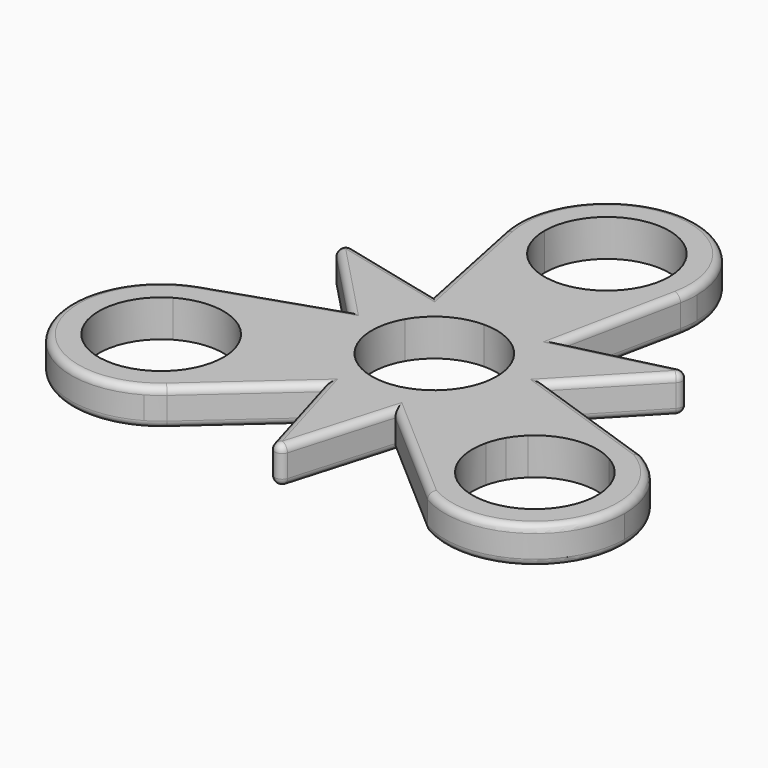
from build123d import *

# Parameters (mm, degrees)
F1_DEPTH      = 6.5278
F2_T3_ANGLE   = 203.1236625431
F2_T6_DEPTH   = 24.7868945093
F2_T10_DEPTH  = 28.7612147001
F2_T14_DEPTH  = 28.7612147001
F2_T18_DEPTH  = 24.7868937804
F2_T22_ANGLE  = 203.1236592361
F2_T25_DEPTH  = 24.7868960458
F2_T29_DEPTH  = 28.7612147001
F2_T33_DEPTH  = 28.8510148795
F2_T37_DEPTH  = 33.4056274337
F2_T41_ANGLE  = 202.9551687841
F2_T44_DEPTH  = 33.4056274337
F2_T48_DEPTH  = 28.8510148795
F2_T52_DEPTH  = 28.7612147001
F2_T56_DEPTH  = 24.7868944005
F2_T60_DEPTH  = 24.7868945093
F2_T64_ANGLE  = 203.1236625431
F2_T67_DEPTH  = 24.7868944005
F2_T71_DEPTH  = 28.7612147001
F2_T75_DEPTH  = 28.8510148795
F2_T79_DEPTH  = 33.4056274337
F2_T83_DEPTH  = 33.4056274337
F2_T87_ANGLE  = 202.9551687841
F2_T90_DEPTH  = 28.8510148795
F2_T94_DEPTH  = 28.7612147001
F2_T98_DEPTH  = 24.7868960458
F2_T102_ANGLE = 203.1236592361
F2_T105_DEPTH = 28.7612147001
F2_T109_DEPTH = 28.7612147001
F2_T113_DEPTH = 24.7868937804
F2_T118_DEPTH = 24.7868945093
F2_T122_DEPTH = 28.7612147001
F2_T128_DEPTH = 28.7612147001
F2_T132_DEPTH = 24.7868937804
F2_T138_DEPTH = 24.7868960458
F2_T142_DEPTH = 28.7612147001
F2_T148_DEPTH = 28.8510148795
F2_T152_DEPTH = 33.4056274337
F2_T158_DEPTH = 33.4056274337
F2_T162_DEPTH = 28.8510148795
F2_T168_DEPTH = 28.7612147001
F2_T172_DEPTH = 24.7868944005
F2_T178_DEPTH = 24.7868945093
F2_T182_DEPTH = 28.7612147001
F2_T188_DEPTH = 28.7612147001
F2_T192_DEPTH = 24.7868944005
F2_T198_DEPTH = 33.4056274337
F2_T202_DEPTH = 28.8510148795
F2_T208_DEPTH = 28.8510148795
F2_T212_DEPTH = 33.4056274337
F2_T218_DEPTH = 24.7868960458
F2_T222_DEPTH = 28.7612147001
F2_T228_DEPTH = 28.7612147001
F2_T232_DEPTH = 24.7868937804
F3_T1_DEPTH   = 3.9878
F3_T6_DEPTH   = 1.27
F3_T12_DEPTH  = 1.27
F3_T18_DEPTH  = 1.27
F3_T24_DEPTH  = 1.27
F3_T30_DEPTH  = 1.27
F3_T36_DEPTH  = 1.27


# Not quite as in the source:
# - a fillet or chamfer that OpenCascade refuses, or shapes differently, is made with other operations: its cross-section is extruded or revolved along the edge and cut away or added
# - a feature names something its author has since deleted; it is built from what else it names


with BuildPart() as f1:
    # F0 (on Top) → F1 (new body)
    with BuildSketch(Plane.XY):
        with BuildLine():
            ThreePointArc((-9.5357191185, 5.50545), (-5.50545, 9.5357191185), (0, 11.0109))
            Line((0, 11.0109), (-7.397765026, 12.8133048875))
            Line((-7.397765026, 12.8133048875), (-9.5357191185, 5.50545))
        make_face()
        with BuildLine():
            Line((-32.9955678842, 19.05), (-13.7481532851, 7.9375))
            ThreePointArc((-13.7481532851, 7.9375), (-12.4088537844, 9.9013116685), (-10.7913433943, 11.6431324285))
            Line((-10.7913433943, 11.6431324285), (-11.2213112334, 13.7448806198))
            Line((-11.2213112334, 13.7448806198), (-32.9955678842, 19.05))
        make_face()
        with BuildLine():
            ThreePointArc((-15.4789201598, 3.5240113062), (-14.7792143279, 5.7957267749), (-13.7481532851, 7.9375))
            Line((-13.7481532851, 7.9375), (-32.9955678842, 19.05))
            Line((-32.9955678842, 19.05), (-17.5140714054, 2.8455002819))
            Line((-17.5140714054, 2.8455002819), (-15.4789201598, 3.5240113062))
        make_face()
        with BuildLine():
            Line((-15.4789201598, 3.5240113062), (-9.5357191185, 5.50545))
            Line((-9.5357191185, 5.50545), (-13.7481532851, 7.9375))
            ThreePointArc((-13.7481532851, 7.9375), (-14.7792143279, 5.7957267749), (-15.4789201598, 3.5240113062))
        make_face()
        with BuildLine():
            Line((-14.795530052, 0), (-9.5357191185, 5.50545))
            Line((-9.5357191185, 5.50545), (-15.4789201598, 3.5240113062))
            ThreePointArc((-15.4789201598, 3.5240113062), (-15.7054057137, 2.3142723193), (-15.8374924179, 1.0906231763))
            Line((-15.8374924179, 1.0906231763), (-14.795530052, 0))
        make_face()
        with BuildLine():
            ThreePointArc((-9.5357191185, -5.50545), (-11.0109, 0), (-9.5357191185, 5.50545))
            Line((-9.5357191185, 5.50545), (-14.795530052, 0))
            Line((-14.795530052, 0), (-9.5357191185, -5.50545))
        make_face()
        with BuildLine():
            Line((-13.7481532851, 7.9375), (-9.5357191185, 5.50545))
            Line((-9.5357191185, 5.50545), (-10.7913433943, 11.6431324285))
            ThreePointArc((-10.7913433943, 11.6431324285), (-12.4088537844, 9.9013116685), (-13.7481532851, 7.9375))
        make_face()
        with BuildLine():
            Line((-11.2213112334, 13.7448806198), (-10.7913433943, 11.6431324285))
            ThreePointArc((-10.7913433943, 11.6431324285), (-9.8569214766, 12.4441441652), (-8.8632535856, 13.170359178))
            Line((-8.8632535856, 13.170359178), (-11.2213112334, 13.7448806198))
        make_face()
        with BuildLine():
            Line((-10.7913433943, 11.6431324285), (-9.5357191185, 5.50545))
            Line((-9.5357191185, 5.50545), (-7.397765026, 12.8133048875))
            Line((-7.397765026, 12.8133048875), (-8.8632535856, 13.170359178))
            ThreePointArc((-8.8632535856, 13.170359178), (-9.8569214766, 12.4441441652), (-10.7913433943, 11.6431324285))
        make_face()
        with BuildLine():
            ThreePointArc((-8.8632535856, 13.170359178), (-7.9375, 13.7481532851), (-6.9742388323, 14.2609823543))
            Line((-6.9742388323, 14.2609823543), (-4.4574811793, 22.863645891))
            ThreePointArc((-4.4574811793, 22.863645891), (-11.6804109204, 27.3490174528), (-15.5528801368, 34.9182482102))
            Line((-15.5528801368, 34.9182482102), (-11.2213112334, 13.7448806198))
            Line((-11.2213112334, 13.7448806198), (-8.8632535856, 13.170359178))
        make_face()
        with BuildLine():
            ThreePointArc((-6.9742388323, 14.2609823543), (-3.5792827581, 15.4662328942), (0, 15.875))
            Line((0, 15.875), (0, 22.225))
            ThreePointArc((0, 22.225), (-2.2514998911, 22.3854725416), (-4.4574811793, 22.863645891))
            Line((-4.4574811793, 22.863645891), (-6.9742388323, 14.2609823543))
        make_face()
        with BuildLine():
            Line((0, 15.875), (0, 11.0109))
            Line((0, 11.0109), (7.397765026, 12.8133048875))
            Line((7.397765026, 12.8133048875), (6.9742388323, 14.2609823543))
            ThreePointArc((6.9742388323, 14.2609823543), (3.5792827581, 15.4662328942), (0, 15.875))
        make_face()
        with BuildLine():
            Line((-7.397765026, 12.8133048875), (0, 11.0109))
            Line((0, 11.0109), (0, 15.875))
            ThreePointArc((0, 15.875), (-3.5792827581, 15.4662328942), (-6.9742388323, 14.2609823543))
            Line((-6.9742388323, 14.2609823543), (-7.397765026, 12.8133048875))
        make_face()
        with BuildLine():
            Line((-8.8632535856, 13.170359178), (-7.397765026, 12.8133048875))
            Line((-7.397765026, 12.8133048875), (-6.9742388323, 14.2609823543))
            ThreePointArc((-6.9742388323, 14.2609823543), (-7.9375, 13.7481532851), (-8.8632535856, 13.170359178))
        make_face()
        with BuildLine():
            ThreePointArc((-15.8374924179, 1.0906231763), (-15.7054057137, 2.3142723193), (-15.4789201598, 3.5240113062))
            Line((-15.4789201598, 3.5240113062), (-17.5140714054, 2.8455002819))
            Line((-17.5140714054, 2.8455002819), (-15.8374924179, 1.0906231763))
        make_face()
        with BuildLine():
            ThreePointArc((-15.8374924179, -1.0906231763), (-15.875, 0), (-15.8374924179, 1.0906231763))
            Line((-15.8374924179, 1.0906231763), (-17.5140714054, 2.8455002819))
            Line((-17.5140714054, 2.8455002819), (-38.0165293825, -3.9899345741))
            ThreePointArc((-38.0165293825, -3.9899345741), (-29.5251489872, -3.5589762224), (-22.0292387544, -7.5715310073))
            Line((-22.0292387544, -7.5715310073), (-15.8374924179, -1.0906231763))
        make_face()
        with BuildLine():
            Line((-13.7481532851, -7.9375), (-9.5357191185, -5.50545))
            Line((-9.5357191185, -5.50545), (-14.795530052, 0))
            Line((-14.795530052, 0), (-15.8374924179, -1.0906231763))
            ThreePointArc((-15.8374924179, -1.0906231763), (-15.1837919663, -4.6333666512), (-13.7481532851, -7.9375))
        make_face()
        with BuildLine():
            Line((-15.8374924179, -1.0906231763), (-14.795530052, 0))
            Line((-14.795530052, 0), (-15.8374924179, 1.0906231763))
            ThreePointArc((-15.8374924179, 1.0906231763), (-15.875, 0), (-15.8374924179, -1.0906231763))
        make_face()
        with BuildLine():
            Line((-19.2474145991, -11.1125), (-13.7481532851, -7.9375))
            ThreePointArc((-13.7481532851, -7.9375), (-15.1837919663, -4.6333666512), (-15.8374924179, -1.0906231763))
            Line((-15.8374924179, -1.0906231763), (-22.0292387544, -7.5715310073))
            ThreePointArc((-22.0292387544, -7.5715310073), (-20.5121378423, -9.2428801685), (-19.2474145991, -11.1125))
        make_face()
        with BuildLine():
            Line((-4.6875767655, -15.1671437346), (0, -11.0109))
            Line((0, -11.0109), (-7.397765026, -12.8133048875))
            Line((-7.397765026, -12.8133048875), (-6.9742388323, -14.2609823543))
            ThreePointArc((-6.9742388323, -14.2609823543), (-5.8484842371, -14.7584164845), (-4.6875767655, -15.1671437346))
        make_face()
        with BuildLine():
            Line((0, -15.875), (0, -11.0109))
            Line((0, -11.0109), (-4.6875767655, -15.1671437346))
            ThreePointArc((-4.6875767655, -15.1671437346), (-2.3703605435, -15.6970384434), (0, -15.875))
        make_face()
        with BuildLine():
            Line((4.7557678685, -15.1459003358), (0, -11.0109))
            Line((0, -11.0109), (0, -15.875))
            ThreePointArc((0, -15.875), (2.4056659337, -15.6916664639), (4.7557678685, -15.1459003358))
        make_face()
        with BuildLine():
            Line((7.397765026, -12.8133048875), (0, -11.0109))
            Line((0, -11.0109), (4.7557678685, -15.1459003358))
            ThreePointArc((4.7557678685, -15.1459003358), (5.8816693428, -14.7452226413), (6.9742388323, -14.2609823543))
            Line((6.9742388323, -14.2609823543), (7.397765026, -12.8133048875))
        make_face()
        with BuildLine():
            Line((8.8632535856, -13.170359178), (7.397765026, -12.8133048875))
            Line((7.397765026, -12.8133048875), (6.9742388323, -14.2609823543))
            ThreePointArc((6.9742388323, -14.2609823543), (7.9375, -13.7481532851), (8.8632535856, -13.170359178))
        make_face()
        with BuildLine():
            Line((-6.9742388323, -14.2609823543), (-7.397765026, -12.8133048875))
            Line((-7.397765026, -12.8133048875), (-8.8632535856, -13.170359178))
            ThreePointArc((-8.8632535856, -13.170359178), (-7.9375, -13.7481532851), (-6.9742388323, -14.2609823543))
        make_face()
        with BuildLine():
            Line((-7.397765026, -12.8133048875), (0, -11.0109))
            ThreePointArc((0, -11.0109), (-5.50545, -9.5357191185), (-9.5357191185, -5.50545))
            Line((-9.5357191185, -5.50545), (-7.397765026, -12.8133048875))
        make_face()
        with BuildLine():
            Line((-7.397765026, -12.8133048875), (-9.5357191185, -5.50545))
            Line((-9.5357191185, -5.50545), (-13.7481532851, -7.9375))
            ThreePointArc((-13.7481532851, -7.9375), (-11.6045092082, -10.832866243), (-8.8632535856, -13.170359178))
            Line((-8.8632535856, -13.170359178), (-7.397765026, -12.8133048875))
        make_face()
        with BuildLine():
            Line((10.7913433943, 11.6431324285), (9.5357191185, 5.50545))
            Line((9.5357191185, 5.50545), (13.7481532851, 7.9375))
            ThreePointArc((13.7481532851, 7.9375), (12.4088537844, 9.9013116685), (10.7913433943, 11.6431324285))
        make_face()
        with BuildLine():
            Line((13.7481532851, 7.9375), (9.5357191185, 5.50545))
            Line((9.5357191185, 5.50545), (15.4946183882, 3.4543343793))
            ThreePointArc((15.4946183882, 3.4543343793), (14.7922147523, 5.7624654203), (13.7481532851, 7.9375))
        make_face()
        with BuildLine():
            Line((15.4946183882, 3.4543343793), (9.5357191185, 5.50545))
            Line((9.5357191185, 5.50545), (14.795530052, 0))
            Line((14.795530052, 0), (15.8374924179, 1.0906231763))
            ThreePointArc((15.8374924179, 1.0906231763), (15.7105720632, 2.2789362531), (15.4946183882, 3.4543343793))
        make_face()
        with BuildLine():
            ThreePointArc((9.5357191185, 5.50545), (10.6357126807, 2.8498306237), (11.0109, 0))
            ThreePointArc((11.0109, 0), (10.6357126807, -2.8498306237), (9.5357191185, -5.50545))
            Line((9.5357191185, -5.50545), (14.795530052, 0))
            Line((14.795530052, 0), (9.5357191185, 5.50545))
        make_face()
        with BuildLine():
            Line((14.795530052, 0), (9.5357191185, -5.50545))
            Line((9.5357191185, -5.50545), (13.7481532851, -7.9375))
            ThreePointArc((13.7481532851, -7.9375), (15.1837919663, -4.6333666512), (15.8374924179, -1.0906231763))
            Line((15.8374924179, -1.0906231763), (14.795530052, 0))
        make_face()
        with BuildLine():
            Line((13.7481532851, -7.9375), (9.5357191185, -5.50545))
            Line((9.5357191185, -5.50545), (7.397765026, -12.8133048875))
            Line((7.397765026, -12.8133048875), (8.8632535856, -13.170359178))
            ThreePointArc((8.8632535856, -13.170359178), (11.6045092082, -10.832866243), (13.7481532851, -7.9375))
        make_face()
        with BuildLine():
            Line((7.397765026, -12.8133048875), (9.5357191185, -5.50545))
            ThreePointArc((9.5357191185, -5.50545), (5.50545, -9.5357191185), (0, -11.0109))
            Line((0, -11.0109), (7.397765026, -12.8133048875))
        make_face()
        with BuildLine():
            Line((15.8374924179, 1.0906231763), (14.795530052, 0))
            Line((14.795530052, 0), (15.8374924179, -1.0906231763))
            ThreePointArc((15.8374924179, -1.0906231763), (15.8656203335, -0.5456339733), (15.875, 0))
            ThreePointArc((15.875, 0), (15.8656203335, 0.5456339733), (15.8374924179, 1.0906231763))
        make_face()
        with BuildLine():
            Line((6.9742388323, 14.2609823543), (7.397765026, 12.8133048875))
            Line((7.397765026, 12.8133048875), (8.8632535856, 13.170359178))
            ThreePointArc((8.8632535856, 13.170359178), (7.9375, 13.7481532851), (6.9742388323, 14.2609823543))
        make_face()
        with BuildLine():
            Line((7.397765026, 12.8133048875), (9.5357191185, 5.50545))
            Line((9.5357191185, 5.50545), (10.7913433943, 11.6431324285))
            ThreePointArc((10.7913433943, 11.6431324285), (9.8569214766, 12.4441441652), (8.8632535856, 13.170359178))
            Line((8.8632535856, 13.170359178), (7.397765026, 12.8133048875))
        make_face()
        with BuildLine():
            ThreePointArc((0, 11.0109), (5.50545, 9.5357191185), (9.5357191185, 5.50545))
            Line((9.5357191185, 5.50545), (7.397765026, 12.8133048875))
            Line((7.397765026, 12.8133048875), (0, 11.0109))
        make_face()
        with BuildLine():
            ThreePointArc((10.7913433943, 11.6431324285), (12.4088537844, 9.9013116685), (13.7481532851, 7.9375))
            Line((13.7481532851, 7.9375), (32.9955678842, 19.05))
            Line((32.9955678842, 19.05), (11.2213112334, 13.7448806198))
            Line((11.2213112334, 13.7448806198), (10.7913433943, 11.6431324285))
        make_face()
        with BuildLine():
            Line((32.9955678842, 19.05), (13.7481532851, 7.9375))
            ThreePointArc((13.7481532851, 7.9375), (14.7922147523, 5.7624654203), (15.4946183882, 3.4543343793))
            Line((15.4946183882, 3.4543343793), (17.4520381252, 2.780569978))
            Line((17.4520381252, 2.780569978), (32.9955678842, 19.05))
        make_face()
        with BuildLine():
            ThreePointArc((8.8632535856, 13.170359178), (9.8569214766, 12.4441441652), (10.7913433943, 11.6431324285))
            Line((10.7913433943, 11.6431324285), (11.2213112334, 13.7448806198))
            Line((11.2213112334, 13.7448806198), (8.8632535856, 13.170359178))
        make_face()
        with BuildLine():
            Line((17.4520381252, 2.780569978), (15.4946183882, 3.4543343793))
            ThreePointArc((15.4946183882, 3.4543343793), (15.7105720632, 2.2789362531), (15.8374924179, 1.0906231763))
            Line((15.8374924179, 1.0906231763), (17.4520381252, 2.780569978))
        make_face()
        with BuildLine():
            ThreePointArc((15.8374924179, -1.0906231763), (15.1837919663, -4.6333666512), (13.7481532851, -7.9375))
            Line((13.7481532851, -7.9375), (19.2474145991, -11.1125))
            ThreePointArc((19.2474145991, -11.1125), (20.5121378423, -9.2428801685), (22.0292387544, -7.5715310073))
            Line((22.0292387544, -7.5715310073), (15.8374924179, -1.0906231763))
        make_face()
        with BuildLine():
            Line((19.2474145991, -11.1125), (13.7481532851, -7.9375))
            ThreePointArc((13.7481532851, -7.9375), (11.6045092082, -10.832866243), (8.8632535856, -13.170359178))
            Line((8.8632535856, -13.170359178), (17.571757575, -15.2921148837))
            ThreePointArc((17.571757575, -15.2921148837), (18.2606379512, -13.1425923731), (19.2474145991, -11.1125))
        make_face()
        with BuildLine():
            Line((17.571757575, -15.2921148837), (8.8632535856, -13.170359178))
            ThreePointArc((8.8632535856, -13.170359178), (7.9375, -13.7481532851), (6.9742388323, -14.2609823543))
            Line((6.9742388323, -14.2609823543), (6.3179748247, -16.5041933533))
            Line((6.3179748247, -16.5041933533), (20.4838505518, -28.8210058026))
            ThreePointArc((20.4838505518, -28.8210058026), (17.4760270235, -22.3905802599), (17.571757575, -15.2921148837))
        make_face()
        with BuildLine():
            ThreePointArc((22.0292387544, -7.5715310073), (20.5121378423, -9.2428801685), (19.2474145991, -11.1125))
            Line((19.2474145991, -11.1125), (23.4598487657, -13.54455))
            ThreePointArc((23.4598487657, -13.54455), (24.3370608071, -12.2477816849), (25.3893219998, -11.0885339067))
            Line((25.3893219998, -11.0885339067), (22.0292387544, -7.5715310073))
        make_face()
        with BuildLine():
            Line((23.4598487657, -13.54455), (19.2474145991, -11.1125))
            ThreePointArc((19.2474145991, -11.1125), (18.2606379512, -13.1425923731), (17.571757575, -15.2921148837))
            Line((17.571757575, -15.2921148837), (22.2976130538, -16.4435308833))
            ThreePointArc((22.2976130538, -16.4435308833), (22.7754204827, -14.95262207), (23.4598487657, -13.54455))
        make_face()
        with BuildLine():
            Line((22.2976130538, -16.4435308833), (17.571757575, -15.2921148837))
            ThreePointArc((17.571757575, -15.2921148837), (17.4760270235, -22.3905802599), (20.4838505518, -28.8210058026))
            Line((20.4838505518, -28.8210058026), (25.0580678842, -32.7981532851))
            Line((25.0580678842, -32.7981532851), (27.4901178842, -28.5857191185))
            ThreePointArc((27.4901178842, -28.5857191185), (22.8715486325, -23.3794518129), (22.2976130538, -16.4435308833))
        make_face()
        with BuildLine():
            ThreePointArc((4.7557678685, -15.1459003358), (2.4056659337, -15.6916664639), (0, -15.875))
            Line((0, -15.875), (0, -38.1))
            Line((0, -38.1), (6.3179748247, -16.5041933533))
            Line((6.3179748247, -16.5041933533), (4.7557678685, -15.1459003358))
        make_face()
        with BuildLine():
            Line((0, -38.1), (0, -15.875))
            ThreePointArc((0, -15.875), (-2.3703605435, -15.6970384434), (-4.6875767655, -15.1671437346))
            Line((-4.6875767655, -15.1671437346), (-6.2927601721, -16.5903809018))
            Line((-6.2927601721, -16.5903809018), (0, -38.1))
        make_face()
        with BuildLine():
            Line((-6.2927601721, -16.5903809018), (-4.6875767655, -15.1671437346))
            ThreePointArc((-4.6875767655, -15.1671437346), (-5.8484842371, -14.7584164845), (-6.9742388323, -14.2609823543))
            Line((-6.9742388323, -14.2609823543), (-6.2927601721, -16.5903809018))
        make_face()
        with BuildLine():
            ThreePointArc((6.9742388323, -14.2609823543), (5.8816693428, -14.7452226413), (4.7557678685, -15.1459003358))
            Line((4.7557678685, -15.1459003358), (6.3179748247, -16.5041933533))
            Line((6.3179748247, -16.5041933533), (6.9742388323, -14.2609823543))
        make_face()
        with BuildLine():
            ThreePointArc((15.875, 0), (15.8656203335, -0.5456339733), (15.8374924179, -1.0906231763))
            Line((15.8374924179, -1.0906231763), (22.0292387544, -7.5715310073))
            ThreePointArc((22.0292387544, -7.5715310073), (28.1288248223, -3.9393932296), (35.2016484635, -3.3290320439))
            Line((35.2016484635, -3.3290320439), (17.4520381252, 2.780569978))
            Line((17.4520381252, 2.780569978), (15.8374924179, 1.0906231763))
            ThreePointArc((15.8374924179, 1.0906231763), (15.8656203335, 0.5456339733), (15.875, 0))
        make_face()
        with BuildLine():
            ThreePointArc((-8.8632535856, -13.170359178), (-11.6045092082, -10.832866243), (-13.7481532851, -7.9375))
            Line((-13.7481532851, -7.9375), (-19.2474145991, -11.1125))
            ThreePointArc((-19.2474145991, -11.1125), (-18.2606379512, -13.1425923731), (-17.571757575, -15.2921148837))
            Line((-17.571757575, -15.2921148837), (-8.8632535856, -13.170359178))
        make_face()
        with BuildLine():
            Line((-6.2927601721, -16.5903809018), (-6.9742388323, -14.2609823543))
            ThreePointArc((-6.9742388323, -14.2609823543), (-7.9375, -13.7481532851), (-8.8632535856, -13.170359178))
            Line((-8.8632535856, -13.170359178), (-17.571757575, -15.2921148837))
            ThreePointArc((-17.571757575, -15.2921148837), (-17.2337689123, -17.1575629017), (-17.1205678842, -19.05))
            ThreePointArc((-17.1205678842, -19.05), (-18.5178297294, -25.5623515662), (-22.4636510869, -30.9283144249))
            Line((-22.4636510869, -30.9283144249), (-6.2927601721, -16.5903809018))
        make_face()
        with BuildLine():
            ThreePointArc((-17.571757575, -15.2921148837), (-18.2606379512, -13.1425923731), (-19.2474145991, -11.1125))
            Line((-19.2474145991, -11.1125), (-23.4598487657, -13.54455))
            ThreePointArc((-23.4598487657, -13.54455), (-22.7754204827, -14.95262207), (-22.2976130538, -16.4435308833))
            Line((-22.2976130538, -16.4435308833), (-17.571757575, -15.2921148837))
        make_face()
        with BuildLine():
            Line((-23.4598487657, -13.54455), (-19.2474145991, -11.1125))
            ThreePointArc((-19.2474145991, -11.1125), (-20.5121378423, -9.2428801685), (-22.0292387544, -7.5715310073))
            Line((-22.0292387544, -7.5715310073), (-25.3893219998, -11.0885339067))
            ThreePointArc((-25.3893219998, -11.0885339067), (-24.3370608071, -12.2477816849), (-23.4598487657, -13.54455))
        make_face()
        with BuildLine():
            Line((-25.3893219998, -11.0885339067), (-22.0292387544, -7.5715310073))
            ThreePointArc((-22.0292387544, -7.5715310073), (-29.5251489872, -3.5589762224), (-38.0165293825, -3.9899345741))
            ThreePointArc((-38.0165293825, -3.9899345741), (-39.5079184174, -4.5722613806), (-40.9330678842, -5.3018467149))
            Line((-40.9330678842, -5.3018467149), (-38.5010178842, -9.5142808815))
            ThreePointArc((-38.5010178842, -9.5142808815), (-31.6829735128, -8.1176162331), (-25.3893219998, -11.0885339067))
        make_face()
        with BuildLine():
            ThreePointArc((-17.1205678842, -19.05), (-17.2337689123, -17.1575629017), (-17.571757575, -15.2921148837))
            Line((-17.571757575, -15.2921148837), (-22.2976130538, -16.4435308833))
            ThreePointArc((-22.2976130538, -16.4435308833), (-22.0631841173, -17.7374056286), (-21.9846678842, -19.05))
            ThreePointArc((-21.9846678842, -19.05), (-23.4598487657, -24.55545), (-27.4901178842, -28.5857191185))
            Line((-27.4901178842, -28.5857191185), (-25.0580678842, -32.7981532851))
            ThreePointArc((-25.0580678842, -32.7981532851), (-23.7136546359, -31.9287309721), (-22.4636510869, -30.9283144249))
            ThreePointArc((-22.4636510869, -30.9283144249), (-18.5178297294, -25.5623515662), (-17.1205678842, -19.05))
        make_face()
        with BuildLine():
            ThreePointArc((-40.9330678842, -5.3018467149), (-46.7437211693, -26.9875), (-25.0580678842, -32.7981532851))
            Line((-25.0580678842, -32.7981532851), (-27.4901178842, -28.5857191185))
            ThreePointArc((-27.4901178842, -28.5857191185), (-42.5312870027, -24.55545), (-38.5010178842, -9.5142808815))
            Line((-38.5010178842, -9.5142808815), (-40.9330678842, -5.3018467149))
        make_face()
        with BuildLine():
            ThreePointArc((6.9742388323, 14.2609823543), (7.9375, 13.7481532851), (8.8632535856, 13.170359178))
            Line((8.8632535856, 13.170359178), (11.2213112334, 13.7448806198))
            Line((11.2213112334, 13.7448806198), (15.5528801149, 34.9182481036))
            ThreePointArc((15.5528801149, 34.9182481036), (11.6804108835, 27.3490174127), (4.4574811793, 22.863645891))
            Line((4.4574811793, 22.863645891), (6.9742388323, 14.2609823543))
        make_face()
        with BuildLine():
            Line((0, 22.225), (0, 15.875))
            ThreePointArc((0, 15.875), (3.5792827581, 15.4662328942), (6.9742388323, 14.2609823543))
            Line((6.9742388323, 14.2609823543), (4.4574811793, 22.863645891))
            ThreePointArc((4.4574811793, 22.863645891), (2.2514998911, 22.3854725416), (0, 22.225))
        make_face()
        with BuildLine():
            Line((11.0109, 38.1), (15.875, 38.1))
            ThreePointArc((15.875, 38.1), (0, 53.975), (-15.875, 38.1))
            Line((-15.875, 38.1), (-11.0109, 38.1))
            ThreePointArc((-11.0109, 38.1), (0, 49.1109), (11.0109, 38.1))
        make_face()
        with BuildLine():
            Line((3.091708946, 27.53206479), (4.4574811793, 22.863645891))
            ThreePointArc((4.4574811793, 22.863645891), (11.6804108835, 27.3490174127), (15.5528801149, 34.9182481036))
            ThreePointArc((15.5528801149, 34.9182481036), (15.7942647316, 36.5009919989), (15.875, 38.1))
            Line((15.875, 38.1), (11.0109, 38.1))
            ThreePointArc((11.0109, 38.1), (8.8114248803, 31.4970680461), (3.091708946, 27.53206479))
        make_face()
        with BuildLine():
            ThreePointArc((-15.5528801368, 34.9182482102), (-11.6804109204, 27.3490174528), (-4.4574811793, 22.863645891))
            Line((-4.4574811793, 22.863645891), (-3.091708946, 27.53206479))
            ThreePointArc((-3.091708946, 27.53206479), (-8.8114248803, 31.4970680461), (-11.0109, 38.1))
            Line((-11.0109, 38.1), (-15.875, 38.1))
            ThreePointArc((-15.875, 38.1), (-15.7942647371, 36.500992053), (-15.5528801368, 34.9182482102))
        make_face()
        with BuildLine():
            ThreePointArc((-4.4574811793, 22.863645891), (-2.2514998911, 22.3854725416), (0, 22.225))
            Line((0, 22.225), (0, 27.0891))
            ThreePointArc((0, 27.0891), (-1.5616403245, 27.2004037549), (-3.091708946, 27.53206479))
            Line((-3.091708946, 27.53206479), (-4.4574811793, 22.863645891))
        make_face()
        with BuildLine():
            Line((0, 27.0891), (0, 22.225))
            ThreePointArc((0, 22.225), (2.2514998911, 22.3854725416), (4.4574811793, 22.863645891))
            Line((4.4574811793, 22.863645891), (3.091708946, 27.53206479))
            ThreePointArc((3.091708946, 27.53206479), (1.5616403245, 27.2004037549), (0, 27.0891))
        make_face()
        with BuildLine():
            ThreePointArc((35.2016484635, -3.3290320439), (28.1288248223, -3.9393932296), (22.0292387544, -7.5715310073))
            Line((22.0292387544, -7.5715310073), (25.3893219998, -11.0885339067))
            ThreePointArc((25.3893219998, -11.0885339067), (31.6829735128, -8.1176162331), (38.5010178842, -9.5142808815))
            Line((38.5010178842, -9.5142808815), (40.9330678842, -5.3018467149))
            Line((40.9330678842, -5.3018467149), (35.2016484635, -3.3290320439))
        make_face()
        with BuildLine():
            ThreePointArc((48.8705678842, -19.05), (46.7437211693, -11.1125), (40.9330678842, -5.3018467149))
            Line((40.9330678842, -5.3018467149), (38.5010178842, -9.5142808815))
            ThreePointArc((38.5010178842, -9.5142808815), (42.5312870027, -13.54455), (44.0064678842, -19.05))
            ThreePointArc((44.0064678842, -19.05), (38.5010178842, -28.5857191185), (27.4901178842, -28.5857191185))
            Line((27.4901178842, -28.5857191185), (25.0580678842, -32.7981532851))
            ThreePointArc((25.0580678842, -32.7981532851), (40.9330678842, -32.7981532851), (48.8705678842, -19.05))
        make_face()
    extrude(amount=F1_DEPTH)

    # F2: fillet of radius 1.27 on 29 edges, made by hand


with BuildPart() as f2_tool1:
    # F2_s2 → F2_t3 (revolve)
    with BuildSketch(Plane(origin=(7.4812581997, 36.5695112874, 0), x_dir=(0, 0, 1), z_dir=(-0.2004253163, -0.9797089836, 0))):
        with BuildLine():
            ThreePointArc((5.2578, -8.2387954487), (6.1558256121, -7.8668210608), (6.5278, -6.9687954487))
            Line((6.5278, -6.9687954487), (6.5278, -8.2387954487))
            Line((6.5278, -8.2387954487), (5.2578, -8.2387954487))
        make_face()
    revolve(axis=Axis((0, 38.1, 6.5278), (0, 0, 1)), revolution_arc=F2_T3_ANGLE)


with BuildPart() as f2_tool4:
    # F2_s5 → F2_t6 (new body)
    with BuildSketch(Plane(origin=(-7.4812548104, 36.5695113413, 0), x_dir=(0, 0, 1), z_dir=(0.2004252289, -0.9797090015, 0))):
        with BuildLine():
            ThreePointArc((5.2578, 8.23879878), (6.1558256121, 7.8668243921), (6.5278, 6.96879878))
            Line((6.5278, 6.96879878), (6.5278, 8.23879878))
            Line((6.5278, 8.23879878), (5.2578, 8.23879878))
        make_face()
    extrude(amount=F2_T6_DEPTH)

    split(bisect_by=Plane(origin=(2.5323896209, 10.393904, 0), x_dir=(0, 0, 1), z_dir=(0.2367171727, 0.9715786022, 0)), keep=Keep.TOP)


with BuildPart() as f2_tool8:
    # F2_s9 → F2_t10 (new body)
    with BuildSketch(Plane(origin=(-10.6689387925, 2.5993995966, 0), x_dir=(0, 0, 1), z_dir=(-0.9715786022, 0.2367171727, 0))):
        with BuildLine():
            ThreePointArc((5.2578, 10.6979548304), (6.1558256121, 10.3259804425), (6.5278, 9.4279548304))
            Line((6.5278, 9.4279548304), (6.5278, 10.6979548304))
            Line((6.5278, 10.6979548304), (5.2578, 10.6979548304))
        make_face()
    extrude(amount=F2_T10_DEPTH)

    split(bisect_by=Plane(origin=(-8.0716253263, -1.6512631311, 0), x_dir=(0, 0, 1), z_dir=(-0.9797090015, -0.2004252289, 0)), keep=Keep.TOP)


with BuildPart() as f2_tool12:
    # F2_s13 → F2_t14 (new body)
    with BuildSketch(Plane(origin=(-27.4536436121, 28.7357595426, 0), x_dir=(0, 0, 1), z_dir=(0.6907923861, -0.7230531649, 0))):
        with BuildLine():
            ThreePointArc((5.2578, 10.6979548304), (6.1558256121, 10.3259804425), (6.5278, 9.4279548304))
            Line((6.5278, 9.4279548304), (6.5278, 10.6979548304))
            Line((6.5278, 10.6979548304), (5.2578, 10.6979548304))
        make_face()
    extrude(amount=F2_T14_DEPTH)

    split(bisect_by=Plane(origin=(-2.6057768433, 7.815864148, 0), x_dir=(0, 0, 1), z_dir=(-0.316281161, 0.9486654981, 0)), keep=Keep.TOP)


with BuildPart() as f2_tool16:
    # F2_s17 → F2_t18 (new body)
    with BuildSketch(Plane(origin=(-11.8962816058, -3.9661711799, 0), x_dir=(0, 0, 1), z_dir=(-0.9486654981, -0.316281161, 0))):
        with BuildLine():
            ThreePointArc((5.2578, 8.23879878), (6.1558256121, 7.8668243921), (6.5278, 6.96879878))
            Line((6.5278, 6.96879878), (6.5278, 8.23879878))
            Line((6.5278, 8.23879878), (5.2578, 8.23879878))
        make_face()
    extrude(amount=F2_T18_DEPTH)

    split(bisect_by=Plane(origin=(-7.735190098, -7.390065744, 0), x_dir=(0, 0, 1), z_dir=(-0.7230531649, -0.6907923861, 0)), keep=Keep.TOP)


with BuildPart() as f2_tool20:
    # F2_s21 → F2_t22 (revolve)
    with BuildSketch(Plane(origin=(-35.4107550569, -11.8057945129, 0), x_dir=(0, 0, 1), z_dir=(0.9486655386, 0.3162810393, 0))):
        with BuildLine():
            ThreePointArc((5.2578, -8.2387939905), (6.1558256121, -7.8668196027), (6.5278, -6.9687939905))
            Line((6.5278, -6.9687939905), (6.5278, -8.2387939905))
            Line((6.5278, -8.2387939905), (5.2578, -8.2387939905))
        make_face()
    revolve(axis=Axis((-32.9955678842, -19.05, 6.5278), (0, 0, 1)), revolution_arc=F2_T22_ANGLE)


with BuildPart() as f2_tool23:
    # F2_s24 → F2_t25 (new body)
    with BuildSketch(Plane(origin=(-27.92949957, -24.763713408, 0), x_dir=(0, 0, 1), z_dir=(0.7482402692, 0.6634278405, 0))):
        with BuildLine():
            ThreePointArc((5.2578, 8.23879878), (6.1558256121, 7.8668243921), (6.5278, 6.96879878))
            Line((6.5278, 6.96879878), (6.5278, 8.23879878))
            Line((6.5278, 8.23879878), (5.2578, 8.23879878))
        make_face()
    extrude(amount=F2_T25_DEPTH)

    split(bisect_by=Plane(origin=(-10.267579719, -3.003838256, 0), x_dir=(0, 0, 1), z_dir=(-0.9597703376, -0.280786216, 0)), keep=Keep.TOP)


with BuildPart() as f2_tool27:
    # F2_s28 → F2_t29 (new body)
    with BuildSketch(Plane(origin=(3.083323311, -10.539271824, 0), x_dir=(0, 0, 1), z_dir=(0.280786216, -0.9597703376, 0))):
        with BuildLine():
            ThreePointArc((5.2578, 10.6979548304), (6.1558256121, 10.3259804425), (6.5278, 9.4279548304))
            Line((6.5278, 9.4279548304), (6.5278, 10.6979548304))
            Line((6.5278, 10.6979548304), (5.2578, 10.6979548304))
        make_face()
    extrude(amount=F2_T29_DEPTH)

    split(bisect_by=Plane(origin=(5.465848483, -6.1646010169, 0), x_dir=(0, 0, 1), z_dir=(0.6634278405, -0.7482402692, 0)), keep=Keep.TOP)


with BuildPart() as f2_tool31:
    # F2_s32 → F2_t33 (new body)
    with BuildSketch(Plane(origin=(-11.1590759548, -38.1434325658, 0), x_dir=(0, 0, 1), z_dir=(0.280786216, 0.9597703376, 0))):
        with BuildLine():
            ThreePointArc((5.2578, 10.6979548304), (6.1558256121, 10.3259804425), (6.5278, 9.4279548304))
            Line((6.5278, 9.4279548304), (6.5278, 10.6979548304))
            Line((6.5278, 10.6979548304), (5.2578, 10.6979548304))
        make_face()
    extrude(amount=F2_T33_DEPTH)

    split(bisect_by=Plane(origin=(-5.4520316872, -6.2705187449, 0), x_dir=(0, 0, 1), z_dir=(-0.6561380549, -0.7546408768, 0)), keep=Keep.TOP)


with BuildPart() as f2_tool35:
    # F2_s36 → F2_t37 (new body)
    with BuildSketch(Plane(origin=(9.3740217281, -8.150436284, 0), x_dir=(0, 0, 1), z_dir=(0.7546408768, -0.6561380549, 0))):
        with BuildLine():
            ThreePointArc((5.2578, 8.30927523), (6.1558256121, 7.9373008421), (6.5278, 7.03927523))
            Line((6.5278, 7.03927523), (6.5278, 8.30927523))
            Line((6.5278, 8.30927523), (5.2578, 8.30927523))
        make_face()
    extrude(amount=F2_T37_DEPTH)

    split(bisect_by=Plane(origin=(10.267579719, -3.003838256, 0), x_dir=(0, 0, 1), z_dir=(0.9597703376, -0.280786216, 0)), keep=Keep.TOP)


with BuildPart() as f2_tool39:
    # F2_s40 → F2_t41 (revolve)
    with BuildSketch(Plane(origin=(27.9742608572, -24.7300313258, 0), x_dir=(0, 0, 1), z_dir=(-0.7492148978, 0.6623269864, 0))):
        with BuildLine():
            ThreePointArc((5.2578, -8.2936887598), (6.1558256121, -7.9217143719), (6.5278, -7.0236887598))
            Line((6.5278, -7.0236887598), (6.5278, -8.2936887598))
            Line((6.5278, -8.2936887598), (5.2578, -8.2936887598))
        make_face()
    revolve(axis=Axis((32.9955678842, -19.05, 6.5278), (0, 0, 1)), revolution_arc=F2_T41_ANGLE)


with BuildPart() as f2_tool42:
    # F2_s43 → F2_t44 (new body)
    with BuildSketch(Plane(origin=(43.3322756947, -14.9154237277, 0), x_dir=(0, 0, 1), z_dir=(-0.9455526623, 0.3254691426, 0))):
        with BuildLine():
            ThreePointArc((5.2578, 8.30927523), (6.1558256121, 7.9373008421), (6.5278, 7.03927523))
            Line((6.5278, 7.03927523), (6.5278, 8.30927523))
            Line((6.5278, 8.30927523), (5.2578, 8.30927523))
        make_face()
    extrude(amount=F2_T44_DEPTH)

    split(bisect_by=Plane(origin=(7.735190098, -7.390065744, 0), x_dir=(0, 0, 1), z_dir=(0.7230531649, -0.6907923861, 0)), keep=Keep.TOP)


with BuildPart() as f2_tool46:
    # F2_s47 → F2_t48 (new body)
    with BuildSketch(Plane(origin=(7.5235822012, 7.8749419235, 0), x_dir=(0, 0, 1), z_dir=(0.6907923861, 0.7230531649, 0))):
        with BuildLine():
            ThreePointArc((5.2578, 10.6979548304), (6.1558256121, 10.3259804425), (6.5278, 9.4279548304))
            Line((6.5278, 9.4279548304), (6.5278, 10.6979548304))
            Line((6.5278, 10.6979548304), (5.2578, 10.6979548304))
        make_face()
    extrude(amount=F2_T48_DEPTH)

    split(bisect_by=Plane(origin=(2.7044126844, 7.8568573158, 0), x_dir=(0, 0, 1), z_dir=(0.3254691426, 0.9455526623, 0)), keep=Keep.TOP)


with BuildPart() as f2_tool50:
    # F2_s51 → F2_t52 (new body)
    with BuildSketch(Plane(origin=(38.6127195669, 9.4076730232, 0), x_dir=(0, 0, 1), z_dir=(-0.9715786022, -0.2367171727, 0))):
        with BuildLine():
            ThreePointArc((5.2578, 10.6979548304), (6.1558256121, 10.3259804425), (6.5278, 9.4279548304))
            Line((6.5278, 9.4279548304), (6.5278, 10.6979548304))
            Line((6.5278, 10.6979548304), (5.2578, 10.6979548304))
        make_face()
    extrude(amount=F2_T52_DEPTH)

    split(bisect_by=Plane(origin=(8.0716253263, -1.6512631311, 0), x_dir=(0, 0, 1), z_dir=(0.9797090015, -0.2004252289, 0)), keep=Keep.TOP)


with BuildPart() as f2_tool54:
    # F2_s55 → F2_t56 (new body)
    with BuildSketch(Plane(origin=(2.5133358054, 12.2855676712, 0), x_dir=(0, 0, 1), z_dir=(0.2004252289, 0.9797090015, 0))):
        with BuildLine():
            ThreePointArc((5.2578, 8.23879878), (6.1558256121, 7.8668243921), (6.5278, 6.96879878))
            Line((6.5278, 6.96879878), (6.5278, 8.23879878))
            Line((6.5278, 8.23879878), (5.2578, 8.23879878))
        make_face()
    extrude(amount=F2_T56_DEPTH)

    split(bisect_by=Plane(origin=(-2.5323896209, 10.393904, 0), x_dir=(0, 0, 1), z_dir=(-0.2367171727, 0.9715786022, 0)), keep=Keep.TOP)


with BuildPart() as f2_tool58:
    # F2_s59 → F2_t60 (new body)
    with BuildSketch(Plane(origin=(-7.4812548104, 36.5695113413, 0), x_dir=(0, 0, 1), z_dir=(0.2004252289, -0.9797090015, 0))):
        with BuildLine():
            ThreePointArc((1.27, 8.23879878), (0.3719743879, 7.8668243921), (0, 6.96879878))
            Line((0, 6.96879878), (0, 8.23879878))
            Line((0, 8.23879878), (1.27, 8.23879878))
        make_face()
    extrude(amount=F2_T60_DEPTH)

    split(bisect_by=Plane(origin=(2.5323896209, 10.393904, 0), x_dir=(0, 0, 1), z_dir=(0.2367171727, 0.9715786022, 0)), keep=Keep.TOP)


with BuildPart() as f2_tool62:
    # F2_s63 → F2_t64 (revolve)
    with BuildSketch(Plane(origin=(7.4812581997, 36.5695112874, 0), x_dir=(0, 0, 1), z_dir=(-0.2004253163, -0.9797089836, 0))):
        with BuildLine():
            ThreePointArc((1.27, -8.2387954487), (0.3719743879, -7.8668210608), (0, -6.9687954487))
            Line((0, -6.9687954487), (0, -8.2387954487))
            Line((0, -8.2387954487), (1.27, -8.2387954487))
        make_face()
    revolve(axis=Axis((0, 38.1, 0), (0, 0, 1)), revolution_arc=F2_T64_ANGLE)


with BuildPart() as f2_tool65:
    # F2_s66 → F2_t67 (new body)
    with BuildSketch(Plane(origin=(2.5133358054, 12.2855676712, 0), x_dir=(0, 0, 1), z_dir=(0.2004252289, 0.9797090015, 0))):
        with BuildLine():
            ThreePointArc((1.27, 8.23879878), (0.3719743879, 7.8668243921), (0, 6.96879878))
            Line((0, 6.96879878), (0, 8.23879878))
            Line((0, 8.23879878), (1.27, 8.23879878))
        make_face()
    extrude(amount=F2_T67_DEPTH)

    split(bisect_by=Plane(origin=(-2.5323896209, 10.393904, 0), x_dir=(0, 0, 1), z_dir=(-0.2367171727, 0.9715786022, 0)), keep=Keep.TOP)


with BuildPart() as f2_tool69:
    # F2_s70 → F2_t71 (new body)
    with BuildSketch(Plane(origin=(38.6127195669, 9.4076730232, 0), x_dir=(0, 0, 1), z_dir=(-0.9715786022, -0.2367171727, 0))):
        with BuildLine():
            ThreePointArc((1.27, 10.6979548304), (0.3719743879, 10.3259804425), (0, 9.4279548304))
            Line((0, 9.4279548304), (0, 10.6979548304))
            Line((0, 10.6979548304), (1.27, 10.6979548304))
        make_face()
    extrude(amount=F2_T71_DEPTH)

    split(bisect_by=Plane(origin=(8.0716253263, -1.6512631311, 0), x_dir=(0, 0, 1), z_dir=(0.9797090015, -0.2004252289, 0)), keep=Keep.TOP)


with BuildPart() as f2_tool73:
    # F2_s74 → F2_t75 (new body)
    with BuildSketch(Plane(origin=(7.5235822012, 7.8749419235, 0), x_dir=(0, 0, 1), z_dir=(0.6907923861, 0.7230531649, 0))):
        with BuildLine():
            ThreePointArc((1.27, 10.6979548304), (0.3719743879, 10.3259804425), (0, 9.4279548304))
            Line((0, 9.4279548304), (0, 10.6979548304))
            Line((0, 10.6979548304), (1.27, 10.6979548304))
        make_face()
    extrude(amount=F2_T75_DEPTH)

    split(bisect_by=Plane(origin=(2.7044126844, 7.8568573158, 0), x_dir=(0, 0, 1), z_dir=(0.3254691426, 0.9455526623, 0)), keep=Keep.TOP)


with BuildPart() as f2_tool77:
    # F2_s78 → F2_t79 (new body)
    with BuildSketch(Plane(origin=(43.3322756947, -14.9154237277, 0), x_dir=(0, 0, 1), z_dir=(-0.9455526623, 0.3254691426, 0))):
        with BuildLine():
            ThreePointArc((1.27, 8.30927523), (0.3719743879, 7.9373008421), (0, 7.03927523))
            Line((0, 7.03927523), (0, 8.30927523))
            Line((0, 8.30927523), (1.27, 8.30927523))
        make_face()
    extrude(amount=F2_T79_DEPTH)

    split(bisect_by=Plane(origin=(7.735190098, -7.390065744, 0), x_dir=(0, 0, 1), z_dir=(0.7230531649, -0.6907923861, 0)), keep=Keep.TOP)


with BuildPart() as f2_tool81:
    # F2_s82 → F2_t83 (new body)
    with BuildSketch(Plane(origin=(9.3740217281, -8.150436284, 0), x_dir=(0, 0, 1), z_dir=(0.7546408768, -0.6561380549, 0))):
        with BuildLine():
            ThreePointArc((1.27, 8.30927523), (0.3719743879, 7.9373008421), (0, 7.03927523))
            Line((0, 7.03927523), (0, 8.30927523))
            Line((0, 8.30927523), (1.27, 8.30927523))
        make_face()
    extrude(amount=F2_T83_DEPTH)

    split(bisect_by=Plane(origin=(10.267579719, -3.003838256, 0), x_dir=(0, 0, 1), z_dir=(0.9597703376, -0.280786216, 0)), keep=Keep.TOP)


with BuildPart() as f2_tool85:
    # F2_s86 → F2_t87 (revolve)
    with BuildSketch(Plane(origin=(27.9742608572, -24.7300313258, 0), x_dir=(0, 0, 1), z_dir=(-0.7492148978, 0.6623269864, 0))):
        with BuildLine():
            ThreePointArc((1.27, -8.2936887598), (0.3719743879, -7.9217143719), (0, -7.0236887598))
            Line((0, -7.0236887598), (0, -8.2936887598))
            Line((0, -8.2936887598), (1.27, -8.2936887598))
        make_face()
    revolve(axis=Axis((32.9955678842, -19.05, 0), (0, 0, 1)), revolution_arc=F2_T87_ANGLE)


with BuildPart() as f2_tool88:
    # F2_s89 → F2_t90 (new body)
    with BuildSketch(Plane(origin=(-11.1590759548, -38.1434325658, 0), x_dir=(0, 0, 1), z_dir=(0.280786216, 0.9597703376, 0))):
        with BuildLine():
            ThreePointArc((1.27, 10.6979548304), (0.3719743879, 10.3259804425), (0, 9.4279548304))
            Line((0, 9.4279548304), (0, 10.6979548304))
            Line((0, 10.6979548304), (1.27, 10.6979548304))
        make_face()
    extrude(amount=F2_T90_DEPTH)

    split(bisect_by=Plane(origin=(-5.4520316872, -6.2705187449, 0), x_dir=(0, 0, 1), z_dir=(-0.6561380549, -0.7546408768, 0)), keep=Keep.TOP)


with BuildPart() as f2_tool92:
    # F2_s93 → F2_t94 (new body)
    with BuildSketch(Plane(origin=(3.083323311, -10.539271824, 0), x_dir=(0, 0, 1), z_dir=(0.280786216, -0.9597703376, 0))):
        with BuildLine():
            ThreePointArc((1.27, 10.6979548304), (0.3719743879, 10.3259804425), (0, 9.4279548304))
            Line((0, 9.4279548304), (0, 10.6979548304))
            Line((0, 10.6979548304), (1.27, 10.6979548304))
        make_face()
    extrude(amount=F2_T94_DEPTH)

    split(bisect_by=Plane(origin=(5.465848483, -6.1646010169, 0), x_dir=(0, 0, 1), z_dir=(0.6634278405, -0.7482402692, 0)), keep=Keep.TOP)


with BuildPart() as f2_tool96:
    # F2_s97 → F2_t98 (new body)
    with BuildSketch(Plane(origin=(-27.92949957, -24.763713408, 0), x_dir=(0, 0, 1), z_dir=(0.7482402692, 0.6634278405, 0))):
        with BuildLine():
            ThreePointArc((1.27, 8.23879878), (0.3719743879, 7.8668243921), (0, 6.96879878))
            Line((0, 6.96879878), (0, 8.23879878))
            Line((0, 8.23879878), (1.27, 8.23879878))
        make_face()
    extrude(amount=F2_T98_DEPTH)

    split(bisect_by=Plane(origin=(-10.267579719, -3.003838256, 0), x_dir=(0, 0, 1), z_dir=(-0.9597703376, -0.280786216, 0)), keep=Keep.TOP)


with BuildPart() as f2_tool100:
    # F2_s101 → F2_t102 (revolve)
    with BuildSketch(Plane(origin=(-35.4107550569, -11.8057945129, 0), x_dir=(0, 0, 1), z_dir=(0.9486655386, 0.3162810393, 0))):
        with BuildLine():
            ThreePointArc((1.27, -8.2387939905), (0.3719743879, -7.8668196027), (0, -6.9687939905))
            Line((0, -6.9687939905), (0, -8.2387939905))
            Line((0, -8.2387939905), (1.27, -8.2387939905))
        make_face()
    revolve(axis=Axis((-32.9955678842, -19.05, 0), (0, 0, 1)), revolution_arc=F2_T102_ANGLE)


with BuildPart() as f2_tool103:
    # F2_s104 → F2_t105 (new body)
    with BuildSketch(Plane(origin=(-27.4536436121, 28.7357595426, 0), x_dir=(0, 0, 1), z_dir=(0.6907923861, -0.7230531649, 0))):
        with BuildLine():
            ThreePointArc((1.27, 10.6979548304), (0.3719743879, 10.3259804425), (0, 9.4279548304))
            Line((0, 9.4279548304), (0, 10.6979548304))
            Line((0, 10.6979548304), (1.27, 10.6979548304))
        make_face()
    extrude(amount=F2_T105_DEPTH)

    split(bisect_by=Plane(origin=(-2.6057768433, 7.815864148, 0), x_dir=(0, 0, 1), z_dir=(-0.316281161, 0.9486654981, 0)), keep=Keep.TOP)


with BuildPart() as f2_tool107:
    # F2_s108 → F2_t109 (new body)
    with BuildSketch(Plane(origin=(-10.6689387925, 2.5993995966, 0), x_dir=(0, 0, 1), z_dir=(-0.9715786022, 0.2367171727, 0))):
        with BuildLine():
            ThreePointArc((1.27, 10.6979548304), (0.3719743879, 10.3259804425), (0, 9.4279548304))
            Line((0, 9.4279548304), (0, 10.6979548304))
            Line((0, 10.6979548304), (1.27, 10.6979548304))
        make_face()
    extrude(amount=F2_T109_DEPTH)

    split(bisect_by=Plane(origin=(-8.0716253263, -1.6512631311, 0), x_dir=(0, 0, 1), z_dir=(-0.9797090015, -0.2004252289, 0)), keep=Keep.TOP)


with BuildPart() as f2_tool111:
    # F2_s112 → F2_t113 (new body)
    with BuildSketch(Plane(origin=(-11.8962816058, -3.9661711799, 0), x_dir=(0, 0, 1), z_dir=(-0.9486654981, -0.316281161, 0))):
        with BuildLine():
            ThreePointArc((1.27, 8.23879878), (0.3719743879, 7.8668243921), (0, 6.96879878))
            Line((0, 6.96879878), (0, 8.23879878))
            Line((0, 8.23879878), (1.27, 8.23879878))
        make_face()
    extrude(amount=F2_T113_DEPTH)

    split(bisect_by=Plane(origin=(-7.735190098, -7.390065744, 0), x_dir=(0, 0, 1), z_dir=(-0.7230531649, -0.6907923861, 0)), keep=Keep.TOP)


with BuildPart() as f2_tool116:
    # F2_s117 → F2_t118 (new body)
    with BuildSketch(Plane(origin=(-7.4812548104, 36.5695113413, 0), x_dir=(0, 0, 1), z_dir=(0.2004252289, -0.9797090015, 0))):
        with BuildLine():
            ThreePointArc((5.2578, 8.23879878), (6.1558256121, 7.8668243921), (6.5278, 6.96879878))
            Line((6.5278, 6.96879878), (6.5278, 8.23879878))
            Line((6.5278, 8.23879878), (5.2578, 8.23879878))
        make_face()
    extrude(amount=F2_T118_DEPTH)

    split(bisect_by=Plane(origin=(2.5323896209, 10.393904, 0), x_dir=(0, 0, 1), z_dir=(-0.2367171727, -0.9715786022, 0)), keep=Keep.TOP)


with BuildPart() as f2_tool120:
    # F2_s121 → F2_t122 (new body)
    with BuildSketch(Plane(origin=(-10.6689387925, 2.5993995966, 0), x_dir=(0, 0, 1), z_dir=(-0.9715786022, 0.2367171727, 0))):
        with BuildLine():
            ThreePointArc((5.2578, 10.6979548304), (6.1558256121, 10.3259804425), (6.5278, 9.4279548304))
            Line((6.5278, 9.4279548304), (6.5278, 10.6979548304))
            Line((6.5278, 10.6979548304), (5.2578, 10.6979548304))
        make_face()
    extrude(amount=F2_T122_DEPTH)

    split(bisect_by=Plane(origin=(-8.0716253263, -1.6512631311, 0), x_dir=(0, 0, 1), z_dir=(0.9797090015, 0.2004252289, 0)), keep=Keep.TOP)


with BuildPart() as f2_tool116_1:
    add(f2_tool116.part)

    # F2_t124: intersect F2_tool120
    add(f2_tool120.part, mode=Mode.INTERSECT)


with BuildPart() as f2_tool126:
    # F2_s127 → F2_t128 (new body)
    with BuildSketch(Plane(origin=(-27.4536436121, 28.7357595426, 0), x_dir=(0, 0, 1), z_dir=(0.6907923861, -0.7230531649, 0))):
        with BuildLine():
            ThreePointArc((5.2578, 10.6979548304), (6.1558256121, 10.3259804425), (6.5278, 9.4279548304))
            Line((6.5278, 9.4279548304), (6.5278, 10.6979548304))
            Line((6.5278, 10.6979548304), (5.2578, 10.6979548304))
        make_face()
    extrude(amount=F2_T128_DEPTH)

    split(bisect_by=Plane(origin=(-2.6057768433, 7.815864148, 0), x_dir=(0, 0, 1), z_dir=(0.316281161, -0.9486654981, 0)), keep=Keep.TOP)


with BuildPart() as f2_tool130:
    # F2_s131 → F2_t132 (new body)
    with BuildSketch(Plane(origin=(-11.8962816058, -3.9661711799, 0), x_dir=(0, 0, 1), z_dir=(-0.9486654981, -0.316281161, 0))):
        with BuildLine():
            ThreePointArc((5.2578, 8.23879878), (6.1558256121, 7.8668243921), (6.5278, 6.96879878))
            Line((6.5278, 6.96879878), (6.5278, 8.23879878))
            Line((6.5278, 8.23879878), (5.2578, 8.23879878))
        make_face()
    extrude(amount=F2_T132_DEPTH)

    split(bisect_by=Plane(origin=(-7.735190098, -7.390065744, 0), x_dir=(0, 0, 1), z_dir=(0.7230531649, 0.6907923861, 0)), keep=Keep.TOP)


with BuildPart() as f2_tool126_1:
    add(f2_tool126.part)

    # F2_t134: intersect F2_tool130
    add(f2_tool130.part, mode=Mode.INTERSECT)


with BuildPart() as f2_tool136:
    # F2_s137 → F2_t138 (new body)
    with BuildSketch(Plane(origin=(-27.92949957, -24.763713408, 0), x_dir=(0, 0, 1), z_dir=(0.7482402692, 0.6634278405, 0))):
        with BuildLine():
            ThreePointArc((5.2578, 8.23879878), (6.1558256121, 7.8668243921), (6.5278, 6.96879878))
            Line((6.5278, 6.96879878), (6.5278, 8.23879878))
            Line((6.5278, 8.23879878), (5.2578, 8.23879878))
        make_face()
    extrude(amount=F2_T138_DEPTH)

    split(bisect_by=Plane(origin=(-10.267579719, -3.003838256, 0), x_dir=(0, 0, 1), z_dir=(0.9597703376, 0.280786216, 0)), keep=Keep.TOP)


with BuildPart() as f2_tool140:
    # F2_s141 → F2_t142 (new body)
    with BuildSketch(Plane(origin=(3.083323311, -10.539271824, 0), x_dir=(0, 0, 1), z_dir=(0.280786216, -0.9597703376, 0))):
        with BuildLine():
            ThreePointArc((5.2578, 10.6979548304), (6.1558256121, 10.3259804425), (6.5278, 9.4279548304))
            Line((6.5278, 9.4279548304), (6.5278, 10.6979548304))
            Line((6.5278, 10.6979548304), (5.2578, 10.6979548304))
        make_face()
    extrude(amount=F2_T142_DEPTH)

    split(bisect_by=Plane(origin=(5.465848483, -6.1646010169, 0), x_dir=(0, 0, 1), z_dir=(-0.6634278405, 0.7482402692, 0)), keep=Keep.TOP)


with BuildPart() as f2_tool136_1:
    add(f2_tool136.part)

    # F2_t144: intersect F2_tool140
    add(f2_tool140.part, mode=Mode.INTERSECT)


with BuildPart() as f2_tool146:
    # F2_s147 → F2_t148 (new body)
    with BuildSketch(Plane(origin=(-11.1590759548, -38.1434325658, 0), x_dir=(0, 0, 1), z_dir=(0.280786216, 0.9597703376, 0))):
        with BuildLine():
            ThreePointArc((5.2578, 10.6979548304), (6.1558256121, 10.3259804425), (6.5278, 9.4279548304))
            Line((6.5278, 9.4279548304), (6.5278, 10.6979548304))
            Line((6.5278, 10.6979548304), (5.2578, 10.6979548304))
        make_face()
    extrude(amount=F2_T148_DEPTH)

    split(bisect_by=Plane(origin=(-5.4520316872, -6.2705187449, 0), x_dir=(0, 0, 1), z_dir=(0.6561380549, 0.7546408768, 0)), keep=Keep.TOP)


with BuildPart() as f2_tool150:
    # F2_s151 → F2_t152 (new body)
    with BuildSketch(Plane(origin=(9.3740217281, -8.150436284, 0), x_dir=(0, 0, 1), z_dir=(0.7546408768, -0.6561380549, 0))):
        with BuildLine():
            ThreePointArc((5.2578, 8.30927523), (6.1558256121, 7.9373008421), (6.5278, 7.03927523))
            Line((6.5278, 7.03927523), (6.5278, 8.30927523))
            Line((6.5278, 8.30927523), (5.2578, 8.30927523))
        make_face()
    extrude(amount=F2_T152_DEPTH)

    split(bisect_by=Plane(origin=(10.267579719, -3.003838256, 0), x_dir=(0, 0, 1), z_dir=(-0.9597703376, 0.280786216, 0)), keep=Keep.TOP)


with BuildPart() as f2_tool146_1:
    add(f2_tool146.part)

    # F2_t154: intersect F2_tool150
    add(f2_tool150.part, mode=Mode.INTERSECT)


with BuildPart() as f2_tool156:
    # F2_s157 → F2_t158 (new body)
    with BuildSketch(Plane(origin=(43.3322756947, -14.9154237277, 0), x_dir=(0, 0, 1), z_dir=(-0.9455526623, 0.3254691426, 0))):
        with BuildLine():
            ThreePointArc((5.2578, 8.30927523), (6.1558256121, 7.9373008421), (6.5278, 7.03927523))
            Line((6.5278, 7.03927523), (6.5278, 8.30927523))
            Line((6.5278, 8.30927523), (5.2578, 8.30927523))
        make_face()
    extrude(amount=F2_T158_DEPTH)

    split(bisect_by=Plane(origin=(7.735190098, -7.390065744, 0), x_dir=(0, 0, 1), z_dir=(-0.7230531649, 0.6907923861, 0)), keep=Keep.TOP)


with BuildPart() as f2_tool160:
    # F2_s161 → F2_t162 (new body)
    with BuildSketch(Plane(origin=(7.5235822012, 7.8749419235, 0), x_dir=(0, 0, 1), z_dir=(0.6907923861, 0.7230531649, 0))):
        with BuildLine():
            ThreePointArc((5.2578, 10.6979548304), (6.1558256121, 10.3259804425), (6.5278, 9.4279548304))
            Line((6.5278, 9.4279548304), (6.5278, 10.6979548304))
            Line((6.5278, 10.6979548304), (5.2578, 10.6979548304))
        make_face()
    extrude(amount=F2_T162_DEPTH)

    split(bisect_by=Plane(origin=(2.7044126844, 7.8568573158, 0), x_dir=(0, 0, 1), z_dir=(-0.3254691426, -0.9455526623, 0)), keep=Keep.TOP)


with BuildPart() as f2_tool156_1:
    add(f2_tool156.part)

    # F2_t164: intersect F2_tool160
    add(f2_tool160.part, mode=Mode.INTERSECT)


with BuildPart() as f2_tool166:
    # F2_s167 → F2_t168 (new body)
    with BuildSketch(Plane(origin=(38.6127195669, 9.4076730232, 0), x_dir=(0, 0, 1), z_dir=(-0.9715786022, -0.2367171727, 0))):
        with BuildLine():
            ThreePointArc((5.2578, 10.6979548304), (6.1558256121, 10.3259804425), (6.5278, 9.4279548304))
            Line((6.5278, 9.4279548304), (6.5278, 10.6979548304))
            Line((6.5278, 10.6979548304), (5.2578, 10.6979548304))
        make_face()
    extrude(amount=F2_T168_DEPTH)

    split(bisect_by=Plane(origin=(8.0716253263, -1.6512631311, 0), x_dir=(0, 0, 1), z_dir=(-0.9797090015, 0.2004252289, 0)), keep=Keep.TOP)


with BuildPart() as f2_tool170:
    # F2_s171 → F2_t172 (new body)
    with BuildSketch(Plane(origin=(2.5133358054, 12.2855676712, 0), x_dir=(0, 0, 1), z_dir=(0.2004252289, 0.9797090015, 0))):
        with BuildLine():
            ThreePointArc((5.2578, 8.23879878), (6.1558256121, 7.8668243921), (6.5278, 6.96879878))
            Line((6.5278, 6.96879878), (6.5278, 8.23879878))
            Line((6.5278, 8.23879878), (5.2578, 8.23879878))
        make_face()
    extrude(amount=F2_T172_DEPTH)

    split(bisect_by=Plane(origin=(-2.5323896209, 10.393904, 0), x_dir=(0, 0, 1), z_dir=(0.2367171727, -0.9715786022, 0)), keep=Keep.TOP)


with BuildPart() as f2_tool166_1:
    add(f2_tool166.part)

    # F2_t174: intersect F2_tool170
    add(f2_tool170.part, mode=Mode.INTERSECT)


with BuildPart() as f2_tool176:
    # F2_s177 → F2_t178 (new body)
    with BuildSketch(Plane(origin=(-7.4812548104, 36.5695113413, 0), x_dir=(0, 0, 1), z_dir=(0.2004252289, -0.9797090015, 0))):
        with BuildLine():
            ThreePointArc((1.27, 8.23879878), (0.3719743879, 7.8668243921), (0, 6.96879878))
            Line((0, 6.96879878), (0, 8.23879878))
            Line((0, 8.23879878), (1.27, 8.23879878))
        make_face()
    extrude(amount=F2_T178_DEPTH)

    split(bisect_by=Plane(origin=(2.5323896209, 10.393904, 0), x_dir=(0, 0, 1), z_dir=(-0.2367171727, -0.9715786022, 0)), keep=Keep.TOP)


with BuildPart() as f2_tool180:
    # F2_s181 → F2_t182 (new body)
    with BuildSketch(Plane(origin=(-10.6689387925, 2.5993995966, 0), x_dir=(0, 0, 1), z_dir=(-0.9715786022, 0.2367171727, 0))):
        with BuildLine():
            ThreePointArc((1.27, 10.6979548304), (0.3719743879, 10.3259804425), (0, 9.4279548304))
            Line((0, 9.4279548304), (0, 10.6979548304))
            Line((0, 10.6979548304), (1.27, 10.6979548304))
        make_face()
    extrude(amount=F2_T182_DEPTH)

    split(bisect_by=Plane(origin=(-8.0716253263, -1.6512631311, 0), x_dir=(0, 0, 1), z_dir=(0.9797090015, 0.2004252289, 0)), keep=Keep.TOP)


with BuildPart() as f2_tool176_1:
    add(f2_tool176.part)

    # F2_t184: intersect F2_tool180
    add(f2_tool180.part, mode=Mode.INTERSECT)


with BuildPart() as f2_tool186:
    # F2_s187 → F2_t188 (new body)
    with BuildSketch(Plane(origin=(38.6127195669, 9.4076730232, 0), x_dir=(0, 0, 1), z_dir=(-0.9715786022, -0.2367171727, 0))):
        with BuildLine():
            ThreePointArc((1.27, 10.6979548304), (0.3719743879, 10.3259804425), (0, 9.4279548304))
            Line((0, 9.4279548304), (0, 10.6979548304))
            Line((0, 10.6979548304), (1.27, 10.6979548304))
        make_face()
    extrude(amount=F2_T188_DEPTH)

    split(bisect_by=Plane(origin=(8.0716253263, -1.6512631311, 0), x_dir=(0, 0, 1), z_dir=(-0.9797090015, 0.2004252289, 0)), keep=Keep.TOP)


with BuildPart() as f2_tool190:
    # F2_s191 → F2_t192 (new body)
    with BuildSketch(Plane(origin=(2.5133358054, 12.2855676712, 0), x_dir=(0, 0, 1), z_dir=(0.2004252289, 0.9797090015, 0))):
        with BuildLine():
            ThreePointArc((1.27, 8.23879878), (0.3719743879, 7.8668243921), (0, 6.96879878))
            Line((0, 6.96879878), (0, 8.23879878))
            Line((0, 8.23879878), (1.27, 8.23879878))
        make_face()
    extrude(amount=F2_T192_DEPTH)

    split(bisect_by=Plane(origin=(-2.5323896209, 10.393904, 0), x_dir=(0, 0, 1), z_dir=(0.2367171727, -0.9715786022, 0)), keep=Keep.TOP)


with BuildPart() as f2_tool186_1:
    add(f2_tool186.part)

    # F2_t194: intersect F2_tool190
    add(f2_tool190.part, mode=Mode.INTERSECT)


with BuildPart() as f2_tool196:
    # F2_s197 → F2_t198 (new body)
    with BuildSketch(Plane(origin=(43.3322756947, -14.9154237277, 0), x_dir=(0, 0, 1), z_dir=(-0.9455526623, 0.3254691426, 0))):
        with BuildLine():
            ThreePointArc((1.27, 8.30927523), (0.3719743879, 7.9373008421), (0, 7.03927523))
            Line((0, 7.03927523), (0, 8.30927523))
            Line((0, 8.30927523), (1.27, 8.30927523))
        make_face()
    extrude(amount=F2_T198_DEPTH)

    split(bisect_by=Plane(origin=(7.735190098, -7.390065744, 0), x_dir=(0, 0, 1), z_dir=(-0.7230531649, 0.6907923861, 0)), keep=Keep.TOP)


with BuildPart() as f2_tool200:
    # F2_s201 → F2_t202 (new body)
    with BuildSketch(Plane(origin=(7.5235822012, 7.8749419235, 0), x_dir=(0, 0, 1), z_dir=(0.6907923861, 0.7230531649, 0))):
        with BuildLine():
            ThreePointArc((1.27, 10.6979548304), (0.3719743879, 10.3259804425), (0, 9.4279548304))
            Line((0, 9.4279548304), (0, 10.6979548304))
            Line((0, 10.6979548304), (1.27, 10.6979548304))
        make_face()
    extrude(amount=F2_T202_DEPTH)

    split(bisect_by=Plane(origin=(2.7044126844, 7.8568573158, 0), x_dir=(0, 0, 1), z_dir=(-0.3254691426, -0.9455526623, 0)), keep=Keep.TOP)


with BuildPart() as f2_tool196_1:
    add(f2_tool196.part)

    # F2_t204: intersect F2_tool200
    add(f2_tool200.part, mode=Mode.INTERSECT)


with BuildPart() as f2_tool206:
    # F2_s207 → F2_t208 (new body)
    with BuildSketch(Plane(origin=(-11.1590759548, -38.1434325658, 0), x_dir=(0, 0, 1), z_dir=(0.280786216, 0.9597703376, 0))):
        with BuildLine():
            ThreePointArc((1.27, 10.6979548304), (0.3719743879, 10.3259804425), (0, 9.4279548304))
            Line((0, 9.4279548304), (0, 10.6979548304))
            Line((0, 10.6979548304), (1.27, 10.6979548304))
        make_face()
    extrude(amount=F2_T208_DEPTH)

    split(bisect_by=Plane(origin=(-5.4520316872, -6.2705187449, 0), x_dir=(0, 0, 1), z_dir=(0.6561380549, 0.7546408768, 0)), keep=Keep.TOP)


with BuildPart() as f2_tool210:
    # F2_s211 → F2_t212 (new body)
    with BuildSketch(Plane(origin=(9.3740217281, -8.150436284, 0), x_dir=(0, 0, 1), z_dir=(0.7546408768, -0.6561380549, 0))):
        with BuildLine():
            ThreePointArc((1.27, 8.30927523), (0.3719743879, 7.9373008421), (0, 7.03927523))
            Line((0, 7.03927523), (0, 8.30927523))
            Line((0, 8.30927523), (1.27, 8.30927523))
        make_face()
    extrude(amount=F2_T212_DEPTH)

    split(bisect_by=Plane(origin=(10.267579719, -3.003838256, 0), x_dir=(0, 0, 1), z_dir=(-0.9597703376, 0.280786216, 0)), keep=Keep.TOP)


with BuildPart() as f2_tool206_1:
    add(f2_tool206.part)

    # F2_t214: intersect F2_tool210
    add(f2_tool210.part, mode=Mode.INTERSECT)


with BuildPart() as f2_tool216:
    # F2_s217 → F2_t218 (new body)
    with BuildSketch(Plane(origin=(-27.92949957, -24.763713408, 0), x_dir=(0, 0, 1), z_dir=(0.7482402692, 0.6634278405, 0))):
        with BuildLine():
            ThreePointArc((1.27, 8.23879878), (0.3719743879, 7.8668243921), (0, 6.96879878))
            Line((0, 6.96879878), (0, 8.23879878))
            Line((0, 8.23879878), (1.27, 8.23879878))
        make_face()
    extrude(amount=F2_T218_DEPTH)

    split(bisect_by=Plane(origin=(-10.267579719, -3.003838256, 0), x_dir=(0, 0, 1), z_dir=(0.9597703376, 0.280786216, 0)), keep=Keep.TOP)


with BuildPart() as f2_tool220:
    # F2_s221 → F2_t222 (new body)
    with BuildSketch(Plane(origin=(3.083323311, -10.539271824, 0), x_dir=(0, 0, 1), z_dir=(0.280786216, -0.9597703376, 0))):
        with BuildLine():
            ThreePointArc((1.27, 10.6979548304), (0.3719743879, 10.3259804425), (0, 9.4279548304))
            Line((0, 9.4279548304), (0, 10.6979548304))
            Line((0, 10.6979548304), (1.27, 10.6979548304))
        make_face()
    extrude(amount=F2_T222_DEPTH)

    split(bisect_by=Plane(origin=(5.465848483, -6.1646010169, 0), x_dir=(0, 0, 1), z_dir=(-0.6634278405, 0.7482402692, 0)), keep=Keep.TOP)


with BuildPart() as f2_tool216_1:
    add(f2_tool216.part)

    # F2_t224: intersect F2_tool220
    add(f2_tool220.part, mode=Mode.INTERSECT)


with BuildPart() as f2_tool226:
    # F2_s227 → F2_t228 (new body)
    with BuildSketch(Plane(origin=(-27.4536436121, 28.7357595426, 0), x_dir=(0, 0, 1), z_dir=(0.6907923861, -0.7230531649, 0))):
        with BuildLine():
            ThreePointArc((1.27, 10.6979548304), (0.3719743879, 10.3259804425), (0, 9.4279548304))
            Line((0, 9.4279548304), (0, 10.6979548304))
            Line((0, 10.6979548304), (1.27, 10.6979548304))
        make_face()
    extrude(amount=F2_T228_DEPTH)

    split(bisect_by=Plane(origin=(-2.6057768433, 7.815864148, 0), x_dir=(0, 0, 1), z_dir=(0.316281161, -0.9486654981, 0)), keep=Keep.TOP)


with BuildPart() as f2_tool230:
    # F2_s231 → F2_t232 (new body)
    with BuildSketch(Plane(origin=(-11.8962816058, -3.9661711799, 0), x_dir=(0, 0, 1), z_dir=(-0.9486654981, -0.316281161, 0))):
        with BuildLine():
            ThreePointArc((1.27, 8.23879878), (0.3719743879, 7.8668243921), (0, 6.96879878))
            Line((0, 6.96879878), (0, 8.23879878))
            Line((0, 8.23879878), (1.27, 8.23879878))
        make_face()
    extrude(amount=F2_T232_DEPTH)

    split(bisect_by=Plane(origin=(-7.735190098, -7.390065744, 0), x_dir=(0, 0, 1), z_dir=(0.7230531649, 0.6907923861, 0)), keep=Keep.TOP)


with BuildPart() as f2_tool226_1:
    add(f2_tool226.part)

    # F2_t234: intersect F2_tool230
    add(f2_tool230.part, mode=Mode.INTERSECT)


with BuildPart() as f1_1:
    add(f1.part)

    # F2_t235: cut F2_tool1, F2_tool4, F2_tool8, F2_tool12, F2_tool16, F2_tool20, F2_tool23, F2_tool27, F2_tool31, F2_tool35, F2_tool39, F2_tool42, F2_tool46, F2_tool50, F2_tool54, F2_tool58, F2_tool62, F2_tool65, F2_tool69, F2_tool73, F2_tool77, F2_tool81, F2_tool85, F2_tool88, F2_tool92, F2_tool96, F2_tool100, F2_tool103, F2_tool107, F2_tool111, F2_tool116, F2_tool126, F2_tool136, F2_tool146, F2_tool156, F2_tool166, F2_tool176, F2_tool186, F2_tool196, F2_tool206, F2_tool216, F2_tool226
    add([f2_tool1.part, f2_tool4.part, f2_tool8.part, f2_tool12.part, f2_tool16.part, f2_tool20.part, f2_tool23.part, f2_tool27.part, f2_tool31.part, f2_tool35.part, f2_tool39.part, f2_tool42.part, f2_tool46.part, f2_tool50.part, f2_tool54.part, f2_tool58.part, f2_tool62.part, f2_tool65.part, f2_tool69.part, f2_tool73.part, f2_tool77.part, f2_tool81.part, f2_tool85.part, f2_tool88.part, f2_tool92.part, f2_tool96.part, f2_tool100.part, f2_tool103.part, f2_tool107.part, f2_tool111.part, f2_tool116_1.part, f2_tool126_1.part, f2_tool136_1.part, f2_tool146_1.part, f2_tool156_1.part, f2_tool166_1.part, f2_tool176_1.part, f2_tool186_1.part, f2_tool196_1.part, f2_tool206_1.part, f2_tool216_1.part, f2_tool226_1.part], mode=Mode.SUBTRACT)

    # F3: fillet of radius 1.27 on 3 edges, made by hand

    # F3_s2 → F3_t1 (cut)
    with BuildSketch(Plane.XY.offset(1.27)):
        with BuildLine():
            ThreePointArc((28.7778920063, 18.0223977999), (30.1783750784, 17.4234929752), (29.996800335, 15.9111866448))
            Line((29.996800335, 15.9111866448), (32.9955678842, 19.05))
            Line((32.9955678842, 19.05), (28.7778920063, 18.0223977999))
        make_face()
        with BuildLine():
            ThreePointArc((-29.996800335, 15.9111866448), (-30.1783750784, 17.4234929752), (-28.7778920063, 18.0223977999))
            Line((-28.7778920063, 18.0223977999), (-32.9955678842, 19.05))
            Line((-32.9955678842, 19.05), (-29.996800335, 15.9111866448))
        make_face()
        with BuildLine():
            ThreePointArc((1.2189083287, -33.9335844447), (0, -34.8469859504), (-1.2189083287, -33.9335844447))
            Line((-1.2189083287, -33.9335844447), (0, -38.1))
            Line((0, -38.1), (1.2189083287, -33.9335844447))
        make_face()
    extrude(amount=F3_T1_DEPTH, mode=Mode.SUBTRACT)


with BuildPart() as f3_tool4:
    # F3_s5 → F3_t6 (new body)
    with BuildSketch(Plane.XY.offset(1.27)):
        Polygon((0, -33.5769859504), (1.2189083287, -33.9335844447), (0, -38.1), (-1.2189083287, -33.9335844447), align=None)
    extrude(amount=-F3_T6_DEPTH)

    # F3_s7 → F3_t8 (revolve, cut)
    with BuildSketch(Plane(origin=(0, -33.5769859504, 1.27), x_dir=(0, 1, 0), z_dir=(-1, 0, 0))):
        with BuildLine():
            ThreePointArc((0, -1.27), (1.27, 0), (0, 1.27))
            Line((0, 1.27), (0, -1.27))
        make_face()
    revolve(axis=Axis((0, -33.5769859504, 1.27), (0, 0, -1)), mode=Mode.SUBTRACT)


with BuildPart() as f1_2:
    add(f1_1.part)

    # F3_t3: cut F3_tool4
    add(f3_tool4.part, mode=Mode.SUBTRACT)


with BuildPart() as f3_tool10:
    # F3_s11 → F3_t12 (new body)
    with BuildSketch(Plane.XY.offset(5.2578)):
        Polygon((0, -33.5769859504), (1.2189083287, -33.9335844447), (0, -38.1), (-1.2189083287, -33.9335844447), align=None)
    extrude(amount=F3_T12_DEPTH)

    # F3_s13 → F3_t14 (revolve, cut)
    with BuildSketch(Plane(origin=(0, -33.5769859504, 5.2578), x_dir=(0, 1, 0), z_dir=(1, 0, 0))):
        with BuildLine():
            ThreePointArc((0, -1.27), (1.27, 0), (0, 1.27))
            Line((0, 1.27), (0, -1.27))
        make_face()
    revolve(axis=Axis((0, -33.5769859504, 5.2578), (0, 0, 1)), mode=Mode.SUBTRACT)


with BuildPart() as f1_3:
    add(f1_2.part)

    # F3_t9: cut F3_tool10
    add(f3_tool10.part, mode=Mode.SUBTRACT)


with BuildPart() as f3_tool16:
    # F3_s17 → F3_t18 (new body)
    with BuildSketch(Plane.XY.offset(1.27)):
        Polygon((-29.0785228156, 16.7884929752), (-29.996800335, 15.9111866448), (-32.9955678842, 19.05), (-28.7778920063, 18.0223977999), align=None)
    extrude(amount=-F3_T18_DEPTH)

    # F3_s19 → F3_t20 (revolve, cut)
    with BuildSketch(Plane(origin=(-29.0785228156, 16.7884929752, 1.27), x_dir=(0.8660254038, -0.5, 0), z_dir=(0.5, 0.8660254038, 0))):
        with BuildLine():
            ThreePointArc((0, -1.27), (1.27, 0), (0, 1.27))
            Line((0, 1.27), (0, -1.27))
        make_face()
    revolve(axis=Axis((-29.0785228156, 16.7884929752, 1.27), (0, 0, -1)), mode=Mode.SUBTRACT)


with BuildPart() as f1_4:
    add(f1_3.part)

    # F3_t15: cut F3_tool16
    add(f3_tool16.part, mode=Mode.SUBTRACT)


with BuildPart() as f3_tool22:
    # F3_s23 → F3_t24 (new body)
    with BuildSketch(Plane.XY.offset(5.2578)):
        Polygon((-29.0785228156, 16.7884929752), (-29.996800335, 15.9111866448), (-32.9955678842, 19.05), (-28.7778920063, 18.0223977999), align=None)
    extrude(amount=F3_T24_DEPTH)

    # F3_s25 → F3_t26 (revolve, cut)
    with BuildSketch(Plane(origin=(-29.0785228156, 16.7884929752, 5.2578), x_dir=(0.8660254038, -0.5, 0), z_dir=(-0.5, -0.8660254038, 0))):
        with BuildLine():
            ThreePointArc((0, -1.27), (1.27, 0), (0, 1.27))
            Line((0, 1.27), (0, -1.27))
        make_face()
    revolve(axis=Axis((-29.0785228156, 16.7884929752, 5.2578), (0, 0, 1)), mode=Mode.SUBTRACT)


with BuildPart() as f1_5:
    add(f1_4.part)

    # F3_t21: cut F3_tool22
    add(f3_tool22.part, mode=Mode.SUBTRACT)


with BuildPart() as f3_tool28:
    # F3_s29 → F3_t30 (new body)
    with BuildSketch(Plane.XY.offset(1.27)):
        Polygon((29.0785228156, 16.7884929752), (28.7778920063, 18.0223977999), (32.9955678842, 19.05), (29.996800335, 15.9111866448), align=None)
    extrude(amount=-F3_T30_DEPTH)

    # F3_s31 → F3_t32 (revolve, cut)
    with BuildSketch(Plane(origin=(29.0785228156, 16.7884929752, 1.27), x_dir=(-0.8660254038, -0.5, 0), z_dir=(0.5, -0.8660254038, 0))):
        with BuildLine():
            ThreePointArc((0, -1.27), (1.27, 0), (0, 1.27))
            Line((0, 1.27), (0, -1.27))
        make_face()
    revolve(axis=Axis((29.0785228156, 16.7884929752, 1.27), (0, 0, -1)), mode=Mode.SUBTRACT)


with BuildPart() as f1_6:
    add(f1_5.part)

    # F3_t27: cut F3_tool28
    add(f3_tool28.part, mode=Mode.SUBTRACT)


with BuildPart() as f3_tool34:
    # F3_s35 → F3_t36 (new body)
    with BuildSketch(Plane.XY.offset(5.2578)):
        Polygon((29.0785228156, 16.7884929752), (28.7778920063, 18.0223977999), (32.9955678842, 19.05), (29.996800335, 15.9111866448), align=None)
    extrude(amount=F3_T36_DEPTH)

    # F3_s37 → F3_t38 (revolve, cut)
    with BuildSketch(Plane(origin=(29.0785228156, 16.7884929752, 5.2578), x_dir=(-0.8660254038, -0.5, 0), z_dir=(-0.5, 0.8660254038, 0))):
        with BuildLine():
            ThreePointArc((0, -1.27), (1.27, 0), (0, 1.27))
            Line((0, 1.27), (0, -1.27))
        make_face()
    revolve(axis=Axis((29.0785228156, 16.7884929752, 5.2578), (0, 0, 1)), mode=Mode.SUBTRACT)


with BuildPart() as f1_7:
    add(f1_6.part)

    # F3_t33: cut F3_tool34
    add(f3_tool34.part, mode=Mode.SUBTRACT)


solid = f1_7.part
